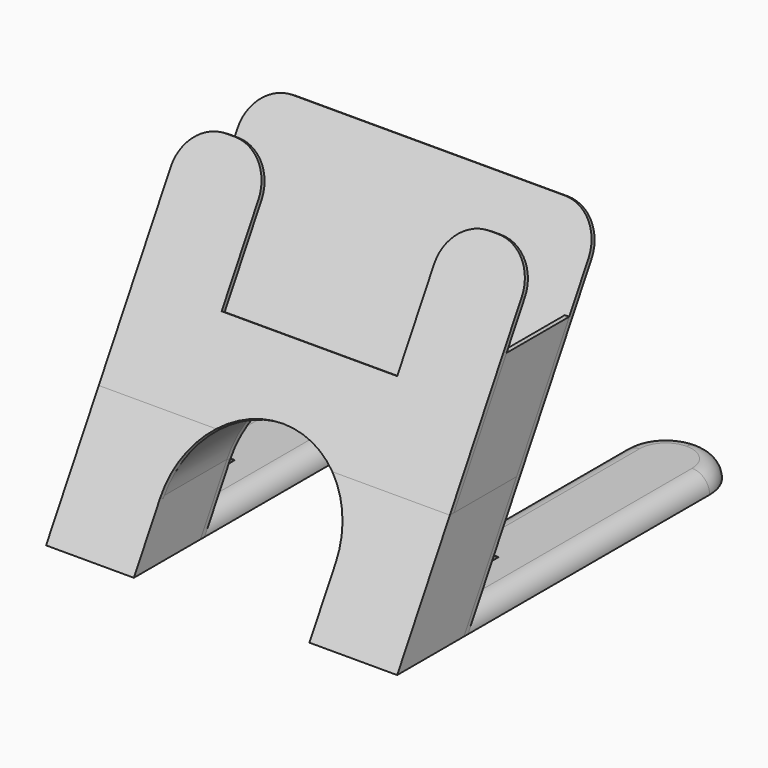
from build123d import *

# Parameters (mm, degrees)
F5_DEPTH    = 4
F6_DEPTH    = 1
F7_DEPTH    = 1
F10_R       = 9
F10_2_R     = 9
F11_R       = 3.99999
F11_2_R     = 3.99999
F15_DEPTH   = 1
F17_DEPTH   = 1
F20_DEPTH   = 0.5
F21_SIZE2   = 0.57734
F21_SIZE    = 0.99999
F22_SIZE2   = 0.57734
F22_SIZE    = 0.99999
F22_2_SIZE2 = 0.57734
F22_2_SIZE  = 0.99999
F22_3_SIZE2 = 0.57734
F22_3_SIZE  = 0.99999
F25_DEPTH   = 0.5


# Not quite as in the source:
# - a fillet or chamfer is up to 0.001 mm smaller than in the source, because OpenCascade refuses the exact size
# - a feature names something its author has since deleted; it is built from what else it names


with BuildPart() as f5:
    # F0 (on Top) → F5 (new body)
    with BuildSketch(Plane.XY):
        with BuildLine():
            Line((20, 39.5), (20, -30.5))
            Line((20, -30.5), (40, -30.5))
            Line((40, -30.5), (40, 39.5))
            ThreePointArc((40, 39.5), (37.0710678119, 46.5710678119), (30, 49.5))
            ThreePointArc((30, 49.5), (22.9289321881, 46.5710678119), (20, 39.5))
        make_face()
    extrude(amount=F5_DEPTH)

    # F11 (radius 4 in the source; OpenCascade refuses exactly that, so slightly less here)
    f11_edges = [f5.edges().sort_by_distance(p)[0] for p in [
        (20, 4.5, 4),
        (40, 4.5, 4),
        (30, 49.5, 4),
    ]]
    fillet(f11_edges, radius=F11_R)


with BuildPart() as f5b:
    # F0 (on Top) → F5, piece 2 (new body)
    with BuildSketch(Plane.XY):
        with BuildLine():
            Line((-40, 39.5), (-40, -30.5))
            Line((-40, -30.5), (-20, -30.5))
            Line((-20, -30.5), (-20, 39.5))
            ThreePointArc((-20, 39.5), (-22.9289321881, 46.5710678119), (-30, 49.5))
            ThreePointArc((-30, 49.5), (-37.0710678119, 46.5710678119), (-40, 39.5))
        make_face()
    extrude(amount=F5_DEPTH)

    # F11#2 (radius 4 in the source; OpenCascade refuses exactly that, so slightly less here)
    f11_2_edges = [f5b.edges().sort_by_distance(p)[0] for p in [
        (-40, 4.5, 4),
        (-20, 4.5, 4),
        (-30, 49.5, 4),
    ]]
    fillet(f11_2_edges, radius=F11_2_R)


with BuildPart() as f6:
    # F4 (on line) → F6 (new body)
    with BuildSketch(Plane(origin=(0, -37.125, 21.4341287437), x_dir=(-1, 0, 0), z_dir=(0, 0.8660254038, -0.5))):
        with BuildLine():
            Line((-40, -24.75), (-20, -24.75))
            Line((-20, -24.75), (-20, -9.75))
            ThreePointArc((-20, -9.75), (-18.2287565553, -1.5212434447), (-13.2287565553, 5.25))
            Line((-13.2287565553, 5.25), (-40, 5.25))
            Line((-40, 5.25), (-40, -24.75))
        make_face()
        with BuildLine():
            Line((13.2287565553, 5.25), (40, 5.25))
            Line((40, 5.25), (40, 55.25))
            Line((40, 55.25), (20, 55.25))
            Line((20, 55.25), (20, 25.25))
            Line((20, 25.25), (-20, 25.25))
            Line((-20, 25.25), (-20, 55.25))
            Line((-20, 55.25), (-40, 55.25))
            Line((-40, 55.25), (-40, 5.25))
            Line((-40, 5.25), (-13.2287565553, 5.25))
            ThreePointArc((-13.2287565553, 5.25), (-7.0710678119, 8.9582869339), (0, 10.25))
            ThreePointArc((0, 10.25), (7.0710678119, 8.9582869339), (13.2287565553, 5.25))
        make_face()
        with BuildLine():
            Line((20, -24.75), (40, -24.75))
            Line((40, -24.75), (40, 5.25))
            Line((40, 5.25), (13.2287565553, 5.25))
            ThreePointArc((13.2287565553, 5.25), (18.2287565553, -1.5212434447), (20, -9.75))
            Line((20, -9.75), (20, -24.75))
        make_face()
    extrude(amount=F6_DEPTH)

    # F10
    f10_edges = [f6.edges().sort_by_distance(p)[0] for p in [
        (-40, -9.066987, 69.032032),
        (-20, -9.066987, 69.032032),
        (40, -9.066987, 69.032032),
        (20, -9.066987, 69.032032),
    ]]
    fillet(f10_edges, radius=F10_R)

    # F22#2 (size 1 and 0.5773502692 in the source; OpenCascade refuses exactly that, so slightly less here)
    f22_2_edges = [f6.edges().sort_by_distance(p)[0] for p in [
        (30, -48.633975, -0.5),
    ]]
    f22_2_side = f6.faces().sort_by_distance((30, -49.066987, -0.25))[0]
    chamfer(f22_2_edges, length=F22_2_SIZE, length2=F22_2_SIZE2, reference=f22_2_side)

    # F22#3 (size 1 and 0.5773502692 in the source; OpenCascade refuses exactly that, so slightly less here)
    f22_3_edges = [f6.edges().sort_by_distance(p)[0] for p in [
        (-30, -48.633975, -0.5),
    ]]
    f22_3_side = f6.faces().sort_by_distance((-30, -49.066987, -0.25))[0]
    chamfer(f22_3_edges, length=F22_3_SIZE, length2=F22_3_SIZE2, reference=f22_3_side)


with BuildPart() as f7:
    # F3 (on line) → F7 (new body)
    with BuildSketch(Plane(origin=(0, -22.875, 13.2068874077), x_dir=(-1, 0, 0), z_dir=(0, 0.8660254038, -0.5))):
        with BuildLine():
            Line((-40, -15.25), (-20, -15.25))
            Line((-20, -15.25), (-20, -0.25))
            ThreePointArc((-20, -0.25), (-18.2287565553, 7.9787565553), (-13.2287565553, 14.75))
            Line((-13.2287565553, 14.75), (-40, 14.75))
            Line((-40, 14.75), (-40, -15.25))
        make_face()
        with BuildLine():
            Line((20, -15.25), (40, -15.25))
            Line((40, -15.25), (40, 14.75))
            Line((40, 14.75), (13.2287565553, 14.75))
            ThreePointArc((13.2287565553, 14.75), (18.2287565553, 7.9787565553), (20, -0.25))
            Line((20, -0.25), (20, -15.25))
        make_face()
        with BuildLine():
            Line((13.2287565553, 14.75), (40, 14.75))
            Line((40, 14.75), (40, 64.75))
            Line((40, 64.75), (-40, 64.75))
            Line((-40, 64.75), (-40, 14.75))
            Line((-40, 14.75), (-13.2287565553, 14.75))
            ThreePointArc((-13.2287565553, 14.75), (-7.0710678119, 18.4582869339), (0, 19.75))
            ThreePointArc((0, 19.75), (7.0710678119, 18.4582869339), (13.2287565553, 14.75))
        make_face()
    extrude(amount=F7_DEPTH)

    # F10#2
    f10_2_edges = [f7.edges().sort_by_distance(p)[0] for p in [
        (40, 9.933013, 69.032032),
        (-40, 9.933013, 69.032032),
    ]]
    fillet(f10_2_edges, radius=F10_2_R)

    # F21 (size 1 and 0.5773502692 in the source; OpenCascade refuses exactly that, so slightly less here)
    f21_edges = [f7.edges().sort_by_distance(p)[0] for p in [
        (30, -29.633975, -0.5),
    ]]
    f21_side = f7.faces().sort_by_distance((30, -30.066987, -0.25))[0]
    chamfer(f21_edges, length=F21_SIZE, length2=F21_SIZE2, reference=f21_side)

    # F22 (size 1 and 0.5773502692 in the source; OpenCascade refuses exactly that, so slightly less here)
    f22_edges = [f7.edges().sort_by_distance(p)[0] for p in [
        (-30, -29.633975, -0.5),
    ]]
    f22_side = f7.faces().sort_by_distance((-30, -30.066987, -0.25))[0]
    chamfer(f22_edges, length=F22_SIZE, length2=F22_SIZE2, reference=f22_side)


with BuildPart() as f8:
    # F4 (on line) → F8 section 0
    with BuildSketch(Plane(origin=(0, -37.125, 21.4341287437), x_dir=(-1, 0, 0), z_dir=(0, 0.8660254038, -0.5))):
        with BuildLine():
            Line((-40, -24.75), (-20, -24.75))
            Line((-20, -24.75), (-20, -9.75))
            ThreePointArc((-20, -9.75), (-18.2287565553, -1.5212434447), (-13.2287565553, 5.25))
            Line((-13.2287565553, 5.25), (-40, 5.25))
            Line((-40, 5.25), (-40, -24.75))
        make_face()
    # F3 (on line) → F8 section 1
    with BuildSketch(Plane(origin=(0, -22.875, 13.2068874077), x_dir=(-1, 0, 0), z_dir=(0, 0.8660254038, -0.5))):
        with BuildLine():
            Line((-40, -15.25), (-20, -15.25))
            Line((-20, -15.25), (-20, -0.25))
            ThreePointArc((-20, -0.25), (-18.2287565553, 7.9787565553), (-13.2287565553, 14.75))
            Line((-13.2287565553, 14.75), (-40, 14.75))
            Line((-40, 14.75), (-40, -15.25))
        make_face()
    loft()


with BuildPart() as f9:
    # F4 (on line) → F9 section 0
    with BuildSketch(Plane(origin=(0, -37.125, 21.4341287437), x_dir=(-1, 0, 0), z_dir=(0, 0.8660254038, -0.5))):
        with BuildLine():
            Line((20, -24.75), (40, -24.75))
            Line((40, -24.75), (40, 5.25))
            Line((40, 5.25), (13.2287565553, 5.25))
            ThreePointArc((13.2287565553, 5.25), (18.2287565553, -1.5212434447), (20, -9.75))
            Line((20, -9.75), (20, -24.75))
        make_face()
    # F3 (on line) → F9 section 1
    with BuildSketch(Plane(origin=(0, -22.875, 13.2068874077), x_dir=(-1, 0, 0), z_dir=(0, 0.8660254038, -0.5))):
        with BuildLine():
            Line((20, -15.25), (40, -15.25))
            Line((40, -15.25), (40, 14.75))
            Line((40, 14.75), (13.2287565553, 14.75))
            ThreePointArc((13.2287565553, 14.75), (18.2287565553, 7.9787565553), (20, -0.25))
            Line((20, -0.25), (20, -15.25))
        make_face()
    loft()


with BuildPart() as f15:
    # F14 (on face) → F15 (new body)
    with BuildSketch(Plane(origin=(-40, 0, 0), x_dir=(0, -1, 0), z_dir=(-1, 0, 0))):
        Polygon((15.5, 25.9807621135), (33.3452994616, 25.9807621135), (18.3452994616, 51.9615242271), (0.5, 51.9615242271), align=None)
    extrude(amount=-F15_DEPTH)


with BuildPart() as f17:
    # F16 (on offset) → F17 (new body)
    with BuildSketch(Plane.YZ.offset(40)):
        Polygon((-18.3452994616, 51.9615242271), (-33.3452994616, 25.9807621135), (-15.5, 25.9807621135), (-0.5, 51.9615242271), align=None)
    extrude(amount=-F17_DEPTH)


with BuildPart() as f20:
    # F19 (on line) → F20 (new body, symmetric)
    with BuildSketch(Plane.YZ.offset(30)):
        Polygon((-22.4594569975, 11.9266290008), (-27.0358983849, 4), (-8.7301328353, 4), align=None)
    extrude(amount=F20_DEPTH, both=True)


with BuildPart() as f25:
    # F24 (on line) → F25 (new body, symmetric)
    with BuildSketch(Plane.YZ.offset(-30)):
        Polygon((-22.4873672427, 11.878287038), (-27.0358983849, 4), (-8.8417738163, 4), align=None)
    extrude(amount=F25_DEPTH, both=True)


solid = Compound([f5.part, f5b.part, f6.part, f7.part, f8.part, f9.part, f15.part, f17.part, f20.part, f25.part])
